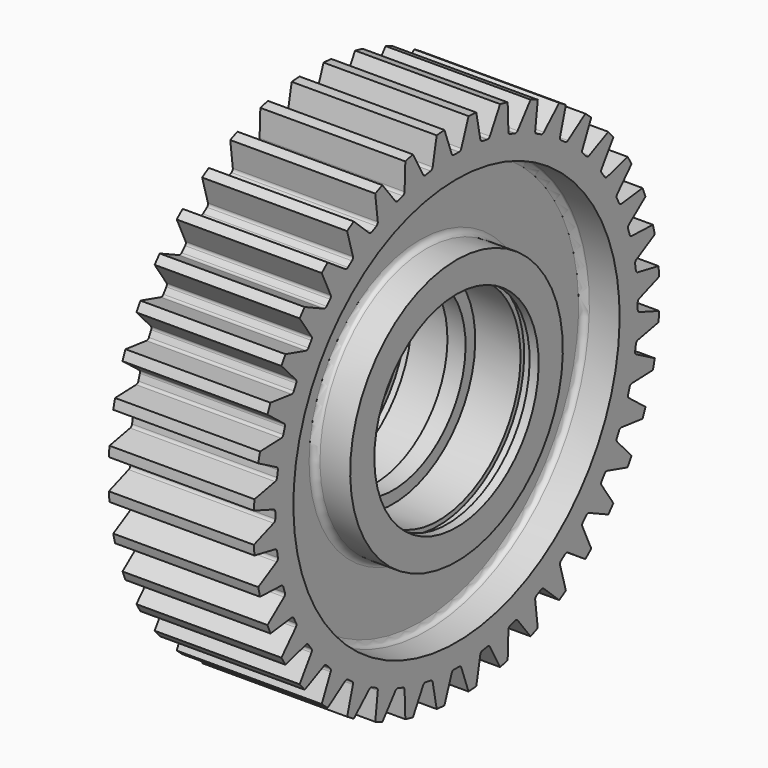
from build123d import *

# Parameters (mm, degrees)
F3_DEPTH = 25
F4_COUNT = 40
F4_ANGLE = 351


with BuildPart() as f1:
    # F0 (on Front) → F1 (revolve)
    with BuildSketch(Plane.XZ):
        with BuildLine():
            Line((24, 84), (0, 84))
            Line((0, 84), (-24, 84))
            Line((-24, 84), (-24, 67.5))
            Line((-24, 67.5), (-14, 67.5))
            ThreePointArc((-14, 67.5), (-12.5857864376, 66.9142135624), (-12, 65.5))
            Line((-12, 65.5), (-12, 46))
            ThreePointArc((-12, 46), (-12.5857864376, 44.5857864376), (-14, 44))
            Line((-14, 44), (-24, 44))
            Line((-24, 44), (-24, 34))
            Line((-24, 34), (-21, 34))
            Line((-21, 34), (-21, 35.5))
            Line((-21, 35.5), (-18, 35.5))
            Line((-18, 35.5), (-18, 34))
            Line((-18, 34), (-3, 34))
            Line((-3, 34), (-3, 30))
            Line((-3, 30), (0, 30))
            Line((0, 30), (3, 30))
            Line((3, 30), (3, 34))
            Line((3, 34), (18, 34))
            Line((18, 34), (18, 35.5))
            Line((18, 35.5), (21, 35.5))
            Line((21, 35.5), (21, 34))
            Line((21, 34), (24, 34))
            Line((24, 34), (24, 44))
            Line((24, 44), (14, 44))
            ThreePointArc((14, 44), (12.5857864376, 44.5857864376), (12, 46))
            Line((12, 46), (12, 65.5))
            ThreePointArc((12, 65.5), (12.5857864376, 66.9142135624), (14, 67.5))
            Line((14, 67.5), (24, 67.5))
            Line((24, 67.5), (24, 84))
        make_face()
    revolve(axis=Axis((-12, 0, 0), (-1, 0, 0)))

    # F2 (on Right) → F3 (cut, symmetric)
    with BuildSketch(Plane.YZ):
        with BuildLine():
            ThreePointArc((-1.0412874443, 74.9927711213), (0, 75), (1.0412874443, 74.9927711213))
            ThreePointArc((1.0412874443, 74.9927711213), (1.6230472701, 75.1695606152), (1.9948638977, 75.650654593))
            Line((1.9948638977, 75.650654593), (4.98, 83.8522486282))
            ThreePointArc((4.98, 83.8522486282), (0, 84), (-4.98, 83.8522486282))
            Line((-4.98, 83.8522486282), (-1.9948638977, 75.650654593))
            ThreePointArc((-1.9948638977, 75.650654593), (-1.6230472701, 75.1695606152), (-1.0412874443, 74.9927711213))
        make_face()
    f3 = extrude(amount=F3_DEPTH, both=True, mode=Mode.SUBTRACT)

    # F4: F3 ×40 about axis
    f4_axis = Axis((24, 0, 0), (-1, 0, 0))
    for i in range(1, F4_COUNT):
        add(f3.rotate(f4_axis, i * F4_ANGLE / (F4_COUNT - 1)), mode=Mode.SUBTRACT)


solid = f1.part
